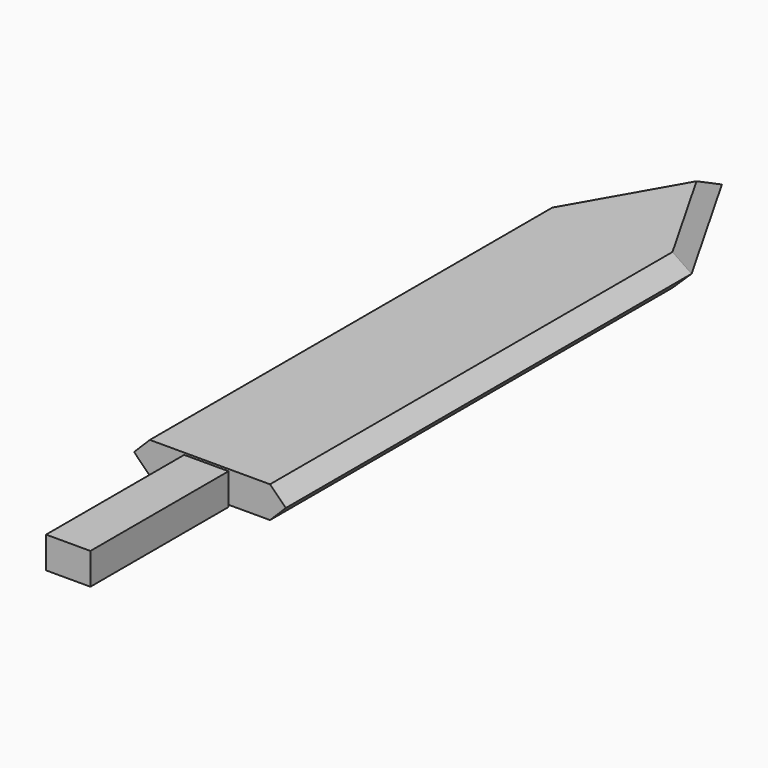
from build123d import *

# Parameters (mm, degrees)
F0_W     = 19.2505270243
F0_H     = 64.3689483404
F1_DEPTH = 4
F2_SIZE  = 2
F3_SIZE  = 1.99999
F4_W     = 5.6250048801
F4_H     = 21.9078958035
F5_DEPTH = 4


# Not quite as in the source:
# - a fillet or chamfer is up to 0.001 mm smaller than in the source, because OpenCascade refuses the exact size


with BuildPart() as f1:
    # F0 (on Top) → F1 (new body)
    with BuildSketch(Plane.XY):
        Polygon((0, 49.0286834538), (-9.6252635121, 32.1844741702), (9.6252635121, 32.1844741702), align=None)
        Rectangle(F0_W, F0_H)
    extrude(amount=F1_DEPTH)

    # F2
    f2_edges = [f1.edges().sort_by_distance(p)[0] for p in [
        (9.625264, 0, 4),
        (4.812632, 40.606579, 4),
        (-4.812632, 40.606579, 4),
        (-9.625264, 0, 4),
    ]]
    chamfer(f2_edges, length=F2_SIZE)

    # F3 (size 2 in the source; OpenCascade refuses exactly that, so slightly less here)
    f3_edges = [f1.edges().sort_by_distance(p)[0] for p in [
        (4.812632, 40.606579, 0),
        (-4.812632, 40.606579, 0),
        (-9.625264, 0, 0),
        (9.625264, 0, 0),
    ]]
    chamfer(f3_edges, length=F3_SIZE)


with BuildPart() as f5:
    # F4 (on Top) → F5 (new body)
    with BuildSketch(Plane.XY):
        with Locations((-0.1480260398, -43.5197390616)):
            Rectangle(F4_W, F4_H)
    extrude(amount=F5_DEPTH)


solid = Compound([f1.part, f5.part])
